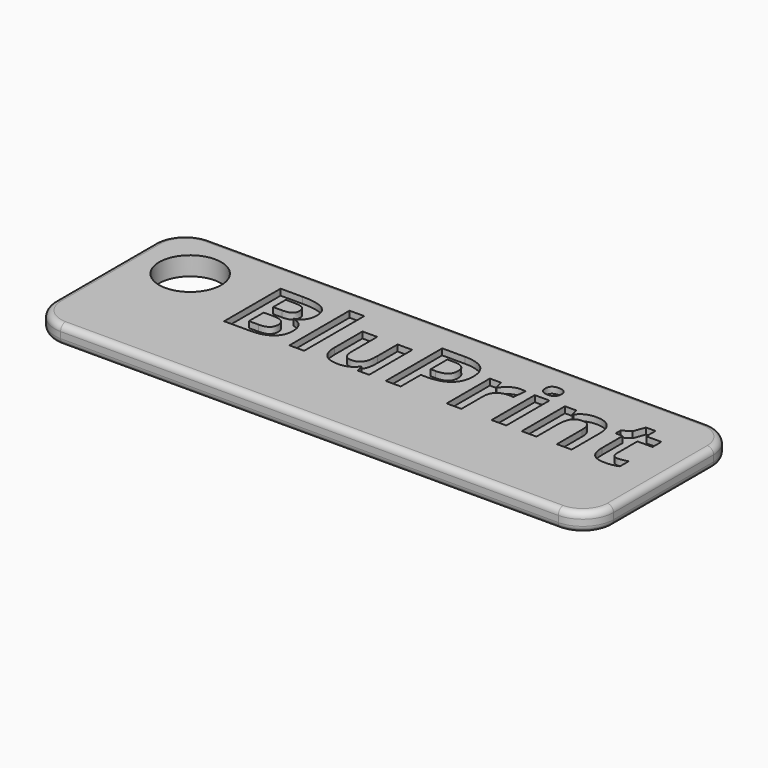
from build123d import *

# Parameters (mm, degrees)
F0_W         = 90
F0_H         = 30
F1_DEPTH     = 3
F2_R         = 1
F3_T1_DEPTH  = 3
F3_T4_ANGLE  = 90
F3_T6_ANGLE  = 90
F3_T8_ANGLE  = 90
F3_T10_ANGLE = 90
F3_T12_ANGLE = 90
F3_T14_ANGLE = 90
F3_T16_ANGLE = 90
F3_T18_ANGLE = 90
F4_R         = 5
F5_DEPTH     = 3
F6_TEXT_SIZE = 15.9215981907
F7_DEPTH     = 1


# Not quite as in the source:
# - a fillet or chamfer that OpenCascade refuses, or shapes differently, is made with other operations: its cross-section is extruded or revolved along the edge and cut away or added
# - Text() gives the source's letters only with a copy of the font that has no kerning and outlines rounded to 1/6400 em; it was checked with that copy


with BuildPart() as f1:
    # F0 (on Top) → F1 (new body)
    with BuildSketch(Plane.XY):
        Rectangle(F0_W, F0_H)
    extrude(amount=F1_DEPTH)

    # F2
    f2_edges = [f1.edges().sort_by_distance(p)[0] for p in [
        (0, 15, 3),
        (-45, 0, 3),
        (0, -15, 3),
        (45, 0, 3),
        (0, 15, 0),
        (-45, 0, 0),
        (0, -15, 0),
        (45, 0, 0),
    ]]
    fillet(f2_edges, radius=F2_R)

    # F3: fillet of radius 5 on 4 edges, made by hand

    # F3_s2 → F3_t1 (cut)
    with BuildSketch(Plane.XY):
        with BuildLine():
            ThreePointArc((45.0004, -9.9990343146), (43.5355339059, -13.5355339059), (39.9990343146, -15.0004))
            Line((39.9990343146, -15.0004), (39.9990343146, -15.5005365685))
            ThreePointArc((39.9990343146, -15.5005365685), (42.4995171573, -15.5001365685), (45, -15.5001365685))
            Line((45, -15.5001365685), (45.5001365685, -15))
            ThreePointArc((45.5001365685, -15), (45.5001365685, -12.4995171573), (45.5005365685, -9.9990343146))
            Line((45.5005365685, -9.9990343146), (45.0004, -9.9990343146))
        make_face()
        with BuildLine():
            ThreePointArc((39.9990343146, 15.0004), (43.5355339059, 13.5355339059), (45.0004, 9.9990343146))
            Line((45.0004, 9.9990343146), (45.5005365685, 9.9990343146))
            ThreePointArc((45.5005365685, 9.9990343146), (45.5001365685, 12.4995171573), (45.5001365685, 15))
            Line((45.5001365685, 15), (45, 15.5001365685))
            ThreePointArc((45, 15.5001365685), (42.4995171573, 15.5001365685), (39.9990343146, 15.5005365685))
            Line((39.9990343146, 15.5005365685), (39.9990343146, 15.0004))
        make_face()
        with BuildLine():
            ThreePointArc((-39.9990343146, 15.0004), (-43.5355339059, 13.5355339059), (-45.0004, 9.9990343146))
            Line((-45.0004, 9.9990343146), (-45.5005365685, 9.9990343146))
            ThreePointArc((-45.5005365685, 9.9990343146), (-45.5001365685, 12.4995171573), (-45.5001365685, 15))
            Line((-45.5001365685, 15), (-45, 15.5001365685))
            ThreePointArc((-45, 15.5001365685), (-42.4995171573, 15.5001365685), (-39.9990343146, 15.5005365685))
            Line((-39.9990343146, 15.5005365685), (-39.9990343146, 15.0004))
        make_face()
        with BuildLine():
            ThreePointArc((-45.0004, -9.9990343146), (-43.5355339059, -13.5355339059), (-39.9990343146, -15.0004))
            Line((-39.9990343146, -15.0004), (-39.9990343146, -15.5005365685))
            ThreePointArc((-39.9990343146, -15.5005365685), (-42.4995171573, -15.5001365685), (-45, -15.5001365685))
            Line((-45, -15.5001365685), (-45.5001365685, -15))
            ThreePointArc((-45.5001365685, -15), (-45.5001365685, -12.4995171573), (-45.5005365685, -9.9990343146))
            Line((-45.5005365685, -9.9990343146), (-45.0004, -9.9990343146))
        make_face()
    extrude(amount=F3_T1_DEPTH, mode=Mode.SUBTRACT)

    # F3_s3 → F3_t4 (revolve, cut)
    with BuildSketch(Plane.YZ.offset(-39.9990343146)):
        with BuildLine():
            ThreePointArc((-14.0004, 0), (-14.7075067812, 0.2928932188), (-15.0004, 1))
            Line((-15.0004, 1), (-15.0004, 0))
            Line((-15.0004, 0), (-14.0004, 0))
        make_face()
    revolve(axis=Axis((-39.9990343146, -9.9990343146, 0), (0, 0, -1)), revolution_arc=F3_T4_ANGLE, mode=Mode.SUBTRACT)

    # F3_s5 → F3_t6 (revolve, cut)
    with BuildSketch(Plane.XZ.offset(9.9990343146)):
        with BuildLine():
            ThreePointArc((-44.0004, 3), (-44.7075067812, 2.7071067812), (-45.0004, 2))
            Line((-45.0004, 2), (-45.0004, 3))
            Line((-45.0004, 3), (-44.0004, 3))
        make_face()
    revolve(axis=Axis((-39.9990343146, -9.9990343146, 3), (0, 0, 1)), revolution_arc=F3_T6_ANGLE, mode=Mode.SUBTRACT)

    # F3_s7 → F3_t8 (revolve, cut)
    with BuildSketch(Plane.XZ.offset(-9.9990343146)):
        with BuildLine():
            ThreePointArc((-44.0004, 0), (-44.7075067812, 0.2928932188), (-45.0004, 1))
            Line((-45.0004, 1), (-45.0004, 0))
            Line((-45.0004, 0), (-44.0004, 0))
        make_face()
    revolve(axis=Axis((-39.9990343146, 9.9990343146, 0), (0, 0, -1)), revolution_arc=F3_T8_ANGLE, mode=Mode.SUBTRACT)

    # F3_s9 → F3_t10 (revolve, cut)
    with BuildSketch(Plane.YZ.offset(-39.9990343146)):
        with BuildLine():
            ThreePointArc((14.0004, 3), (14.7075067812, 2.7071067812), (15.0004, 2))
            Line((15.0004, 2), (15.0004, 3))
            Line((15.0004, 3), (14.0004, 3))
        make_face()
    revolve(axis=Axis((-39.9990343146, 9.9990343146, 3), (0, 0, 1)), revolution_arc=F3_T10_ANGLE, mode=Mode.SUBTRACT)

    # F3_s11 → F3_t12 (revolve, cut)
    with BuildSketch(Plane.YZ.offset(39.9990343146)):
        with BuildLine():
            ThreePointArc((14.0004, 0), (14.7075067812, 0.2928932188), (15.0004, 1))
            Line((15.0004, 1), (15.0004, 0))
            Line((15.0004, 0), (14.0004, 0))
        make_face()
    revolve(axis=Axis((39.9990343146, 9.9990343146, 0), (0, 0, -1)), revolution_arc=F3_T12_ANGLE, mode=Mode.SUBTRACT)

    # F3_s13 → F3_t14 (revolve, cut)
    with BuildSketch(Plane.XZ.offset(-9.9990343146)):
        with BuildLine():
            ThreePointArc((44.0004, 3), (44.7075067812, 2.7071067812), (45.0004, 2))
            Line((45.0004, 2), (45.0004, 3))
            Line((45.0004, 3), (44.0004, 3))
        make_face()
    revolve(axis=Axis((39.9990343146, 9.9990343146, 3), (0, 0, 1)), revolution_arc=F3_T14_ANGLE, mode=Mode.SUBTRACT)

    # F3_s15 → F3_t16 (revolve, cut)
    with BuildSketch(Plane.XZ.offset(9.9990343146)):
        with BuildLine():
            ThreePointArc((44.0004, 0), (44.7075067812, 0.2928932188), (45.0004, 1))
            Line((45.0004, 1), (45.0004, 0))
            Line((45.0004, 0), (44.0004, 0))
        make_face()
    revolve(axis=Axis((39.9990343146, -9.9990343146, 0), (0, 0, -1)), revolution_arc=F3_T16_ANGLE, mode=Mode.SUBTRACT)

    # F3_s17 → F3_t18 (revolve, cut)
    with BuildSketch(Plane.YZ.offset(39.9990343146)):
        with BuildLine():
            ThreePointArc((-14.0004, 3), (-14.7075067812, 2.7071067812), (-15.0004, 2))
            Line((-15.0004, 2), (-15.0004, 3))
            Line((-15.0004, 3), (-14.0004, 3))
        make_face()
    revolve(axis=Axis((39.9990343146, -9.9990343146, 3), (0, 0, 1)), revolution_arc=F3_T18_ANGLE, mode=Mode.SUBTRACT)

    # F4 (on face) → F5 (cut)
    with BuildSketch(Plane.XY.offset(3)):
        with Locations((-36, 6)):
            Circle(F4_R)
    extrude(amount=-F5_DEPTH, mode=Mode.SUBTRACT)

    # F6 (on face) → F7 (cut)
    with BuildSketch(Plane.XY.offset(3)):
        with Locations((-26, -1.4635506973)):
            Text('BluPrint', F6_TEXT_SIZE, font='Open Sans', font_style=FontStyle.BOLD, text_align=(TextAlign.LEFT, TextAlign.BOTTOM))
    extrude(amount=-F7_DEPTH, mode=Mode.SUBTRACT)


solid = f1.part
